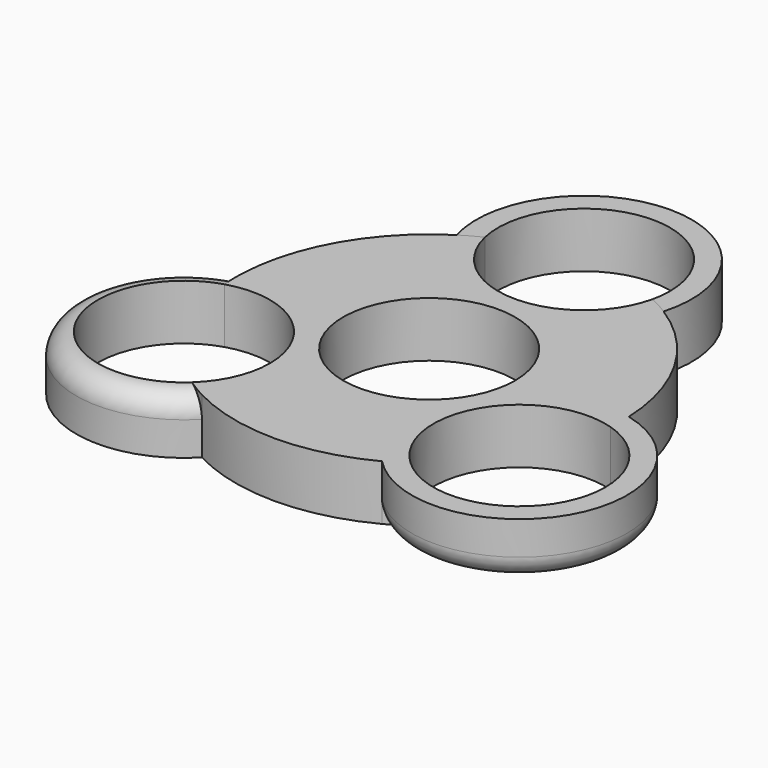
from build123d import *
from build123d import SkipClean  # not in build123d's __all__

# Parameters (mm, degrees)
F0_R         = 11.0744
F1_DEPTH     = 7.112
F3_T3_ANGLE  = 270.1069651298
F3_S4_R      = 24.9492229885
F3_T5_DEPTH  = 22
F3_T8_ANGLE  = 270.1069651298
F3_S9_R      = 24.9492229885
F3_T10_DEPTH = 22


# Not quite as in the source:
# - a fillet or chamfer that OpenCascade refuses, or shapes differently, is made with other operations: its cross-section is extruded or revolved along the edge and cut away or added
# - a feature of the source that left no trace in its solid (it failed there, or was rolled back) is left out
# - a pattern or mirror of a feature is missing from the dataset's text; its kind, count and spacing are read off the source's solid


with BuildPart() as f1:
    # F0 (on Top) → F1 (new body)
    with BuildSketch(Plane.XY):
        with BuildLine():
            ThreePointArc((-10.7982111441, 22.491384213), (-1.236653926, 35.9543591725), (11.0744, 24.9492229885))
            ThreePointArc((11.0744, 24.9492229885), (11.005136184, 23.7125690625), (10.7982111441, 22.491384213))
            ThreePointArc((10.7982111441, 22.491384213), (12.0832280354, 21.8279483226), (13.3276464943, 21.0911727187))
            ThreePointArc((13.3276464943, 21.0911727187), (0, 38.824045977), (-13.3276464943, 21.0911727187))
            ThreePointArc((-13.3276464943, 21.0911727187), (-12.0832280354, 21.8279483226), (-10.7982111441, 22.491384213))
        make_face()
        with BuildLine():
            ThreePointArc((10.7982111441, 22.491384213), (0, 13.8748229885), (-10.7982111441, 22.491384213))
            ThreePointArc((-10.7982111441, 22.491384213), (-12.0832280354, 21.8279483226), (-13.3276464943, 21.0911727187))
            ThreePointArc((-13.3276464943, 21.0911727187), (-12.7649941961, 19.5117938041), (-12.0159491811, 18.0118114943))
            ThreePointArc((-12.0159491811, 18.0118114943), (-12.0159491811, 6.9374114943), (-21.6066609127, 1.4002114943))
            ThreePointArc((-21.6066609127, 1.4002114943), (-23.2802062059, 1.2989123509), (-24.9293146172, 0.9964940774))
            ThreePointArc((-24.9293146172, 0.9964940774), (-24.9451717776, -0.4495917229), (-24.8772156668, -1.8941669402))
            ThreePointArc((-24.8772156668, -1.8941669402), (-15.0331191052, -3.5622109498), (-10.5322609127, -12.4746114943))
            ThreePointArc((-10.5322609127, -12.4746114943), (-11.4576064423, -16.9062058706), (-14.0790045227, -20.5972172728))
            ThreePointArc((-14.0790045227, -20.5972172728), (-12.8619437422, -21.3783565997), (-11.6016681229, -22.0876667961))
            ThreePointArc((-11.6016681229, -22.0876667961), (-10.5152120097, -20.8107061551), (-9.5907117317, -19.4120229885))
            ThreePointArc((-9.5907117317, -19.4120229885), (0, -13.8748229885), (9.5907117317, -19.4120229885))
            ThreePointArc((9.5907117317, -19.4120229885), (10.5152120097, -20.8107061551), (11.6016681229, -22.0876667961))
            ThreePointArc((11.6016681229, -22.0876667961), (12.8619437422, -21.3783565997), (14.0790045227, -20.5972172728))
            ThreePointArc((14.0790045227, -20.5972172728), (12.0159491811, -6.9374114943), (24.8772156668, -1.8941669402))
            ThreePointArc((24.8772156668, -1.8941669402), (24.9312146589, -0.947767568), (24.9492229885, 0))
            ThreePointArc((24.9492229885, 0), (24.9442453991, 0.4983464632), (24.9293146172, 0.9964940774))
            ThreePointArc((24.9293146172, 0.9964940774), (23.2802062059, 1.2989123509), (21.6066609127, 1.4002114943))
            ThreePointArc((21.6066609127, 1.4002114943), (12.0159491811, 6.9374114943), (12.0159491811, 18.0118114943))
            ThreePointArc((12.0159491811, 18.0118114943), (12.7649941961, 19.5117938041), (13.3276464943, 21.0911727187))
            ThreePointArc((13.3276464943, 21.0911727187), (12.0832280354, 21.8279483226), (10.7982111441, 22.491384213))
        make_face()
        Circle(F0_R, mode=Mode.SUBTRACT)
        with BuildLine():
            ThreePointArc((-12.0159491811, 18.0118114943), (-12.7649941961, 19.5117938041), (-13.3276464943, 21.0911727187))
            ThreePointArc((-13.3276464943, 21.0911727187), (-21.6066609127, 12.4746114943), (-24.9293146172, 0.9964940774))
            ThreePointArc((-24.9293146172, 0.9964940774), (-23.2802062059, 1.2989123509), (-21.6066609127, 1.4002114943))
            ThreePointArc((-21.6066609127, 1.4002114943), (-12.0159491811, 6.9374114943), (-12.0159491811, 18.0118114943))
        make_face()
        with BuildLine():
            ThreePointArc((24.9293146172, 0.9964940774), (21.6066609127, 12.4746114943), (13.3276464943, 21.0911727187))
            ThreePointArc((13.3276464943, 21.0911727187), (12.7649941961, 19.5117938041), (12.0159491811, 18.0118114943))
            ThreePointArc((12.0159491811, 18.0118114943), (12.0159491811, 6.9374114943), (21.6066609127, 1.4002114943))
            ThreePointArc((21.6066609127, 1.4002114943), (23.2802062059, 1.2989123509), (24.9293146172, 0.9964940774))
        make_face()
        with BuildLine():
            ThreePointArc((11.6016681229, -22.0876667961), (33.6226100938, -19.4120229885), (24.9293146172, 0.9964940774))
            ThreePointArc((24.9293146172, 0.9964940774), (24.9442453991, 0.4983464632), (24.9492229885, 0))
            ThreePointArc((24.9492229885, 0), (24.9312146589, -0.947767568), (24.8772156668, -1.8941669402))
            ThreePointArc((24.8772156668, -1.8941669402), (30.5190614572, -5.9010696867), (32.6810609127, -12.4746114943))
            ThreePointArc((32.6810609127, -12.4746114943), (26.0382552891, -22.6236659647), (14.0790045227, -20.5972172728))
            ThreePointArc((14.0790045227, -20.5972172728), (12.8619437422, -21.3783565997), (11.6016681229, -22.0876667961))
        make_face()
        with BuildLine():
            ThreePointArc((-9.5907117317, -19.4120229885), (-10.5152120097, -20.8107061551), (-11.6016681229, -22.0876667961))
            ThreePointArc((-11.6016681229, -22.0876667961), (0, -24.9492229885), (11.6016681229, -22.0876667961))
            ThreePointArc((11.6016681229, -22.0876667961), (10.5152120097, -20.8107061551), (9.5907117317, -19.4120229885))
            ThreePointArc((9.5907117317, -19.4120229885), (0, -13.8748229885), (-9.5907117317, -19.4120229885))
        make_face()
    extrude(amount=F1_DEPTH)

    # F1_copies: F1 across plane


with BuildPart() as f1_1:
    add(f1.part, clean=False)
    with SkipClean():  # cleaning this boolean's faces spoils the solid; the shape is the same uncleaned
        add(f1.part.mirror(Plane(origin=(0, 0, 0), x_dir=(-0.8660254038, 0.5, 0), z_dir=(-0.5, -0.8660254038, 0))), clean=False)

    # F3: fillet of radius 2.794 on 2 edges, made by hand


with BuildPart() as f3_tool1:
    # F3_s2 → F3_t3 (revolve)
    with BuildSketch(Plane(origin=(4.5458669208, -17.0289729971, 0), x_dir=(0, 0, 1), z_dir=(-0.2579172921, 0.9661669993, 0))):
        with BuildLine():
            ThreePointArc((0, 6.5774017335), (0.8183436534, 4.6017453869), (2.794, 3.7834017335))
            Line((2.794, 3.7834017335), (0, 3.7834017335))
            Line((0, 3.7834017335), (0, 6.5774017335))
        make_face()
    revolve(axis=Axis((21.6066609127, -12.4746114943, 0), (0, 0, 1)), revolution_arc=F3_T3_ANGLE)

    # F3_s4 → F3_t5 (cut, symmetric)
    with BuildSketch(Plane.XY.offset(2.4)):
        Circle(F3_S4_R)
    extrude(amount=F3_T5_DEPTH, both=True, mode=Mode.SUBTRACT)


with BuildPart() as f3_tool6:
    # F3_s7 → F3_t8 (revolve)
    with BuildSketch(Plane(origin=(-4.5458669208, -17.0289729971, 0), x_dir=(0, 0, 1), z_dir=(0.2579172921, 0.9661669993, 0))):
        with BuildLine():
            ThreePointArc((7.112, -6.5774017335), (6.2936563466, -4.6017453869), (4.318, -3.7834017335))
            Line((4.318, -3.7834017335), (7.112, -3.7834017335))
            Line((7.112, -3.7834017335), (7.112, -6.5774017335))
        make_face()
    revolve(axis=Axis((-21.6066609127, -12.4746114943, 7.112), (0, 0, -1)), revolution_arc=F3_T8_ANGLE)

    # F3_s9 → F3_t10 (cut, symmetric)
    with BuildSketch(Plane.XY.offset(5.7)):
        Circle(F3_S9_R)
    extrude(amount=F3_T10_DEPTH, both=True, mode=Mode.SUBTRACT)


with BuildPart() as f1_2:
    add(f1_1.part, clean=False)

    # F3_t11: cut F3_tool1, F3_tool6
    add([f3_tool1.part, f3_tool6.part], mode=Mode.SUBTRACT)


solid = f1_2.part
